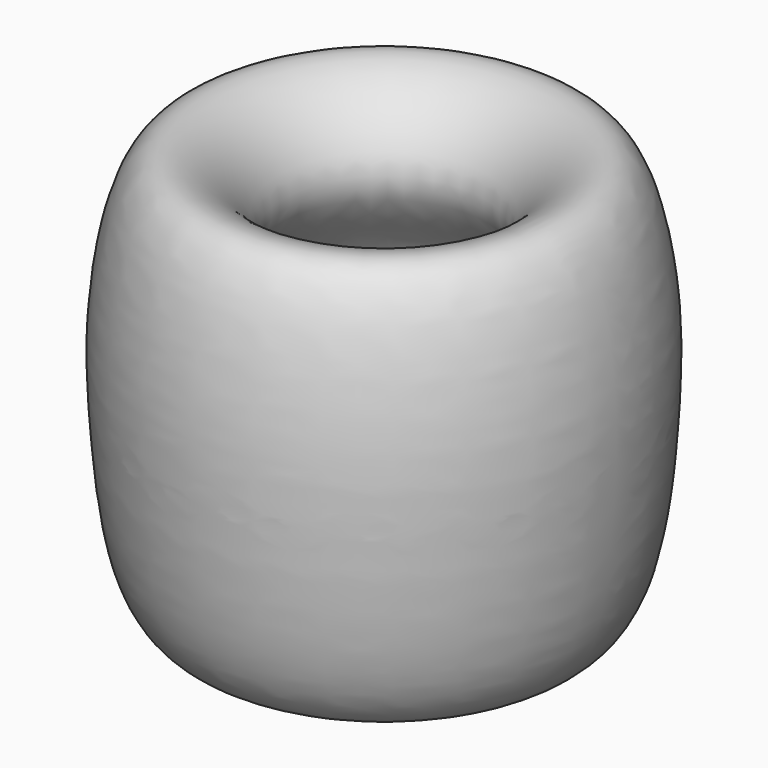
from build123d import *


with BuildPart() as f1:
    # F0 (on Front) → F1 (revolve)
    with BuildSketch(Plane.XZ):
        with BuildLine():
            add(Edge.make_bspline(
                [(0, -12.7373365685), (1.2433632887, -10.5532668522), (13.3748363609, -10.5317322614), (21.285301535, -6.7455465904), (28.0375501441, 14.7447000541), (7.968017381, 27.2448967365), (28.6648476927, 46.5574630012), (34.8047445682, 23.2749711164), (34.5039911056, 6.7119403363), (32.6098596873, -13.3255459599), (27.2663101898, -21.5752524653), (23.4036915269, -22.0428352846), (20.7518320531, -22.1829991788)],
                knots=[0.1566021566, 0.1566021566, 0.1566021566, 0.1566021566, 0.2364129345, 0.3050051701, 0.4023398275, 0.497943931, 0.5876615555, 0.6790488364, 0.7779384558, 0.8780753418, 0.9438805949, 1, 1, 1, 1], degree=3))
            Line((0, -12.7373365685), (0, -14.7471210495))
            add(Edge.make_bspline(
                [(20.7518320531, -22.1829991788), (16.534788255, -22.4058908088), (6.7210949405, -22.4564203234), (0.6722845362, -16.4942791129), (0, -14.7471210495)],
                knots=[0, 0, 0, 0, 0.0892422813, 0.1362649638, 0.1362649638, 0.1362649638, 0.1362649638], degree=3))
        make_face()
    revolve(axis=Axis((0, 0, 0.5724579096), (0, 0, -1)))


solid = f1.part
